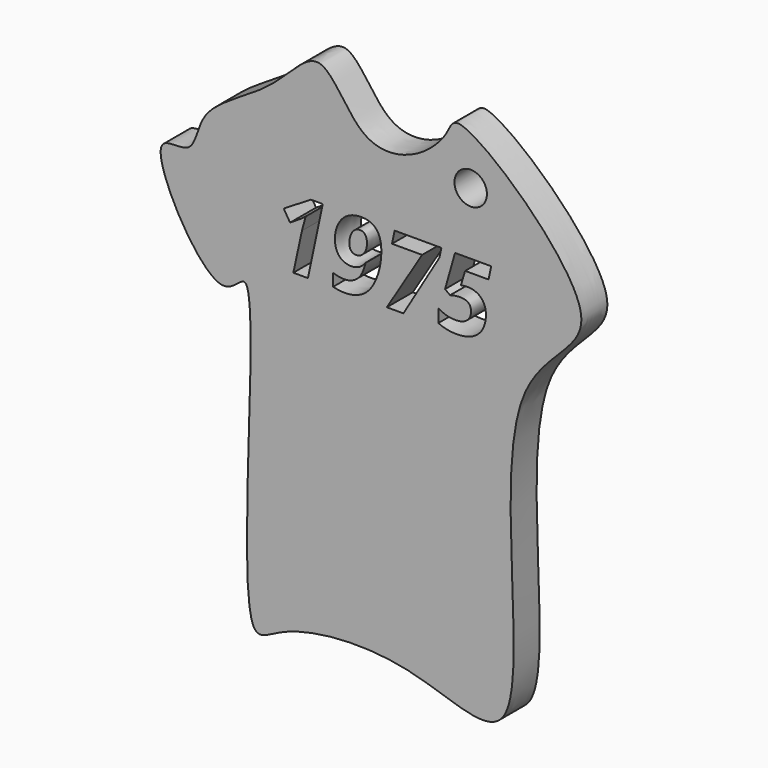
from build123d import *

# Parameters (mm, degrees)
F1_DEPTH     = 5
F4_D         = 5
F2_TEXT_SIZE = 15.1020422992
F5_DEPTH     = 25


# Not quite as in the source:
# - Text() gives the source's letters only with a copy of the font that has no kerning and outlines rounded to 1/6400 em; it was checked with that copy


with BuildPart() as f1:
    # F0 (on Front) → F1 (new body)
    with BuildSketch(Plane.XZ):
        with BuildLine():
            add(Edge.make_bspline(
                [(-40.2171686292, 40.3783433139), (-42.3067699055, 40.8921948791), (-47.3273920844, 33.6600453044), (-59.1278099361, 29.1564222088), (-59.1919739653, 20.8757678023), (-68.7395078236, 24.169635544), (-55.9023824448, 0.2655046896), (-48.2716707367, 15.4682731626), (-54.1253965223, -44.9532990444), (-45.2732174223, -36.8773182533), (-26.5800166534, -35.1517821671), (-4.4538727143, -48.0938703353), (-17.1200010441, 9.9523501547), (9.6203964664, 16.6919215256), (-19.1379037359, 42.3248296952), (-20.3686591508, 36.9223441595), (-25.3830379027, 31.9169775554), (-34.3707161225, 30.9917004244), (-38.0366855041, 39.8421430927), (-40.2171686292, 40.3783433139)],
                knots=[0, 0, 0, 0, 0.0499796957, 0.1090119983, 0.1488234586, 0.1822288553, 0.252995216, 0.2852315465, 0.3973141857, 0.4317535145, 0.5057514748, 0.5680333874, 0.6783900642, 0.7460013113, 0.8317942447, 0.8585741067, 0.9019207494, 0.9478465656, 1, 1, 1, 1], degree=3))
        make_face()
    extrude(amount=F1_DEPTH)

    # F4 (through all)
    with Locations(Plane.XZ.offset(5)):
        with Locations((-16.9426072389, 31.0388524085)):
            Hole(F4_D / 2)

    # F2 (on face) → F5 (cut)
    with BuildSketch(Plane.XZ.offset(5)):
        with Locations((-47.0617450774, 10.7035730034)):
            Text('1975', F2_TEXT_SIZE, font='Open Sans', font_style=FontStyle.BOLDITALIC, text_align=(TextAlign.LEFT, TextAlign.BOTTOM))
    extrude(amount=-F5_DEPTH, mode=Mode.SUBTRACT)


solid = f1.part
